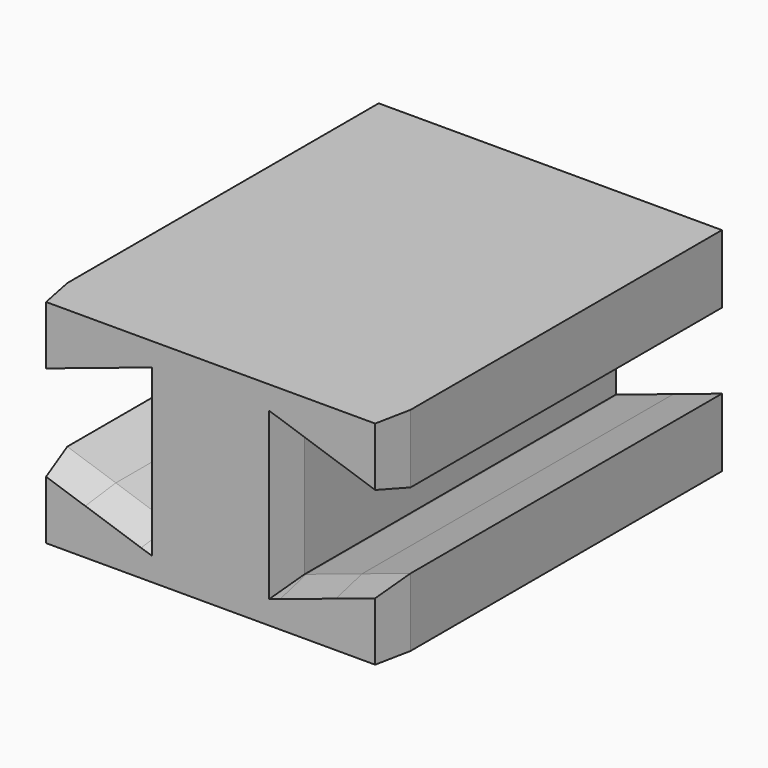
from build123d import *

# Parameters (mm, degrees)
F1_DEPTH = 60
F3_SIZE2 = 5
F3_SIZE  = 1


# Not quite as in the source:
# - a feature names something its author has since deleted; it is built from what else it names


with BuildPart() as f1:
    # F0 (on Front) → F1 (new body)
    with BuildSketch(Plane.XZ):
        Polygon((-9.5, 15), (-24.25, 15), (-24.25, 9.9166666667), (-17.3952847075, 7.6317615692), (-9.5, 10.2635231383), align=None)
        Polygon((-17.3952847075, 7.6317615692), (-24.25, 9.9166666667), (-24.25, 5.3468564717), align=None)
        Polygon((0, 15), (-9.25, 15), (-9.25, 10.3468564717), (-9.25, 4.9166666667), (-9.25, -10.3468564717), (-9.25, -15), (0, -15), align=None)
        Polygon((-9.25, 15), (-9.5, 15), (-9.5, 10.2635231383), (-9.25, 10.3468564717), align=None)
        Polygon((-17.3952847075, -7.6317615692), (-24.25, -9.9166666667), (-24.25, -15), (-9.5, -15), (-9.5, -10.2635231383), align=None)
        Polygon((-24.25, -5.3468564717), (-24.25, -9.9166666667), (-17.3952847075, -7.6317615692), align=None)
        Polygon((-9.25, -10.3468564717), (-9.5, -10.2635231383), (-9.5, -15), (-9.25, -15), align=None)
    extrude(amount=F1_DEPTH)

    # F2: F1 across face


with BuildPart() as f1_1:
    add(f1.part)
    add(f1.part.mirror(Plane(origin=(0, -30, 0), x_dir=(0, 1, 0), z_dir=(1, 0, 0))))

    # F3
    f3_edges = [f1_1.edges().sort_by_distance(p)[0] for p in [
        (-24.25, -60, 10.173428),
        (9.25, -60, 0),
        (16.75, -60, 7.846856),
        (24.25, -60, 10.173428),
        (-16.75, -60, 7.846856),
        (-9.25, -60, 0),
        (-16.75, -60, -7.846856),
        (-24.25, -60, -10.173428),
        (16.75, -60, -7.846856),
        (24.25, -60, -10.173428),
    ]]
    f3_side = f1_1.faces().sort_by_distance((0, -60, 0))[0]
    chamfer(f3_edges, length=F3_SIZE, length2=F3_SIZE2, reference=f3_side)


solid = f1_1.part
